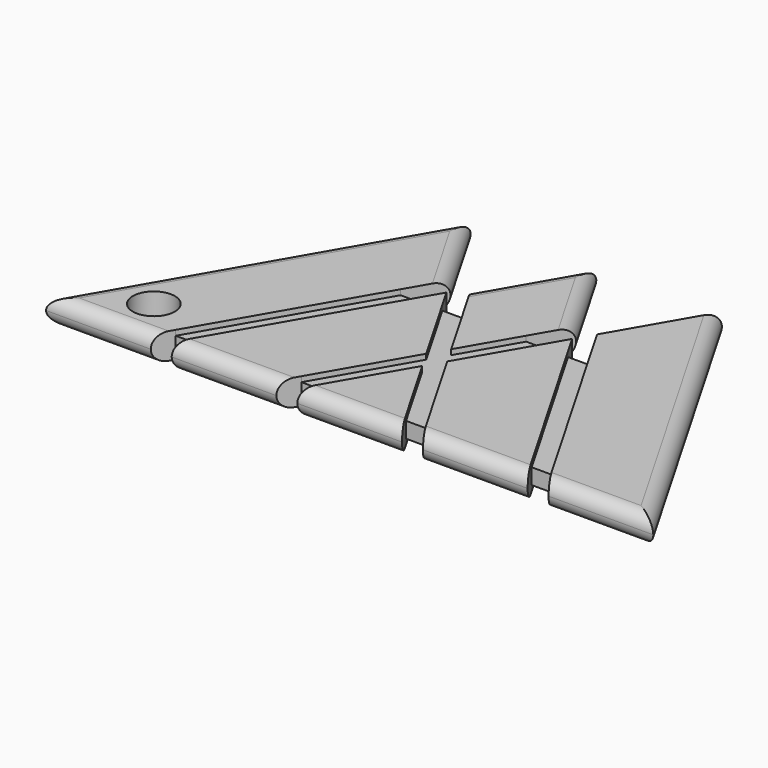
from build123d import *

# Parameters (mm, degrees)
F1_DEPTH = 3.175
F0_R     = 5.1001358677
F2_DEPTH = 1.905
F3_R     = 3.17499
F3_2_R   = 3.17499
F3_3_R   = 3.17499
F3_4_R   = 3.17499
F3_5_R   = 3.17499
F3_6_R   = 3.17499


# Not quite as in the source:
# - a fillet or chamfer is up to 0.001 mm smaller than in the source, because OpenCascade refuses the exact size


with BuildPart() as f1:
    # F0 (on Top) → F1 (new body, symmetric)
    with BuildSketch(Plane.XY):
        Polygon((55.88, 43.9940905122), (33.02, 4.3994090512), (30.48, 0), (55.88, 0), (58.42, 4.3994090512), (71.12, 26.3964543073), (60.96, 43.9940905122), (58.42, 48.3934995635), align=None)
    extrude(amount=F1_DEPTH, both=True)

    # F3#3 (radius 3.175 in the source; OpenCascade refuses exactly that, so slightly less here)
    f3_3_edges = [f1.edges().sort_by_distance(p)[0] for p in [
        (43.18, 0, -3.175),
        (43.18, 0, 3.175),
    ]]
    fillet(f3_3_edges, radius=F3_3_R)


with BuildPart() as f1b:
    # F0 (on Top) → F1, piece 2 (new body, symmetric)
    with BuildSketch(Plane.XY):
        Polygon((60.9602140859, 52.792537807), (66.04, 43.9940905122), (73.6602140859, 30.7954925508), (81.2823551529, 43.9952028573), (86.3618197643, 52.79161069), (73.6618197643, 74.7886559461), align=None)
    extrude(amount=F1_DEPTH, both=True)

    # F3#2 (radius 3.175 in the source; OpenCascade refuses exactly that, so slightly less here)
    f3_2_edges = [f1b.edges().sort_by_distance(p)[0] for p in [
        (67.311017, 63.790597, 3.175),
        (80.01182, 63.790133, 3.175),
        (80.01182, 63.790133, -3.175),
        (67.311017, 63.790597, -3.175),
    ]]
    fillet(f3_2_edges, radius=F3_2_R)


with BuildPart() as f1c:
    # F0 (on Top) → F1, piece 3 (new body, symmetric)
    with BuildSketch(Plane.XY):
        Polygon((88.9005352487, 48.3944264851), (86.360214113, 43.9952028573), (76.1989295703, 26.398308346), (88.9, 4.3994090512), (91.44, 0), (116.84, 0), (114.300072982, 4.3994511866), (91.4404622667, 43.9949752986), align=None)
    extrude(amount=F1_DEPTH, both=True)

    # F3#5 (radius 3.175 in the source; OpenCascade refuses exactly that, so slightly less here)
    f3_5_edges = [f1c.edges().sort_by_distance(p)[0] for p in [
        (104.14, 0, -3.175),
        (104.14, 0, 3.175),
    ]]
    fillet(f3_5_edges, radius=F3_5_R)


with BuildPart() as f1d:
    # F0 (on Top) → F1, piece 4 (new body, symmetric)
    with BuildSketch(Plane.XY):
        Polygon((73.66, 21.9970452561), (63.5, 4.3994090512), (60.96, 0), (86.36, 0), (83.82, 4.3994090512), align=None)
    extrude(amount=F1_DEPTH, both=True)

    # F3#4 (radius 3.175 in the source; OpenCascade refuses exactly that, so slightly less here)
    f3_4_edges = [f1d.edges().sort_by_distance(p)[0] for p in [
        (73.66, 0, -3.175),
        (73.66, 0, 3.175),
    ]]
    fillet(f3_4_edges, radius=F3_4_R)


with BuildPart() as f1e:
    # F0 (on Top) → F1, piece 5 (new body, symmetric)
    with BuildSketch(Plane.XY):
        Polygon((91.4408563844, 52.793650113), (96.520559582, 43.9949752986), (119.3800827134, 4.3994511866), (121.92, 0), (147.32, 0), (104.1424620628, 74.7897682521), align=None)
    extrude(amount=F1_DEPTH, both=True)

    # F3#6 (radius 3.175 in the source; OpenCascade refuses exactly that, so slightly less here)
    f3_6_edges = [f1e.edges().sort_by_distance(p)[0] for p in [
        (134.62, 0, -3.175),
        (125.731231, 37.394884, -3.175),
        (97.791659, 63.791709, -3.175),
        (134.62, 0, 3.175),
        (125.731231, 37.394884, 3.175),
    ]]
    fillet(f3_6_edges, radius=F3_6_R)


with BuildPart() as f1f:
    # F0 (on Top) → F1, piece 6 (new body, symmetric)
    with BuildSketch(Plane.XY):
        Polygon((43.18, 74.7899538708), (0, 0), (25.4, 0), (27.94, 4.3994090512), (50.8, 43.9940905122), (55.88, 52.7929086147), align=None)
        with Locations((18.0367678404, 10.1385600865)):
            Circle(F0_R, mode=Mode.SUBTRACT)
    extrude(amount=F1_DEPTH, both=True)

    # F3 (radius 3.175 in the source; OpenCascade refuses exactly that, so slightly less here)
    f3_edges = [f1f.edges().sort_by_distance(p)[0] for p in [
        (21.59, 37.394977, 3.175),
        (21.59, 37.394977, -3.175),
        (12.7, 0, -3.175),
        (12.7, 0, 3.175),
        (49.53, 63.791431, 3.175),
        (49.53, 63.791431, -3.175),
    ]]
    fillet(f3_edges, radius=F3_R)


with BuildPart() as f2:
    # F0 (on Top) → F2 (new body, symmetric)
    with BuildSketch(Plane.XY):
        Polygon((96.520559582, 43.9949752986), (91.4404622667, 43.9949752986), (114.300072982, 4.3994511866), (119.3800827134, 4.3994511866), align=None)
    extrude(amount=F2_DEPTH, both=True)


with BuildPart() as f2b:
    # F0 (on Top) → F2, piece 2 (new body, symmetric)
    with BuildSketch(Plane.XY):
        Polygon((66.04, 43.9940905122), (60.96, 43.9940905122), (71.12, 26.3964543073), (58.42, 4.3994090512), (63.5, 4.3994090512), (73.66, 21.9970452561), (83.82, 4.3994090512), (88.9, 4.3994090512), (76.1989295703, 26.398308346), (86.360214113, 43.9952028573), (81.2823551529, 43.9952028573), (73.6602140859, 30.7954925508), align=None)
    extrude(amount=F2_DEPTH, both=True)


with BuildPart() as f2c:
    # F0 (on Top) → F2, piece 3 (new body, symmetric)
    with BuildSketch(Plane.XY):
        Polygon((50.8, 43.9940905122), (27.94, 4.3994090512), (33.02, 4.3994090512), (55.88, 43.9940905122), align=None)
    extrude(amount=F2_DEPTH, both=True)


solid = Compound([f1.part, f1b.part, f1c.part, f1d.part, f1e.part, f1f.part, f2.part, f2b.part, f2c.part])
